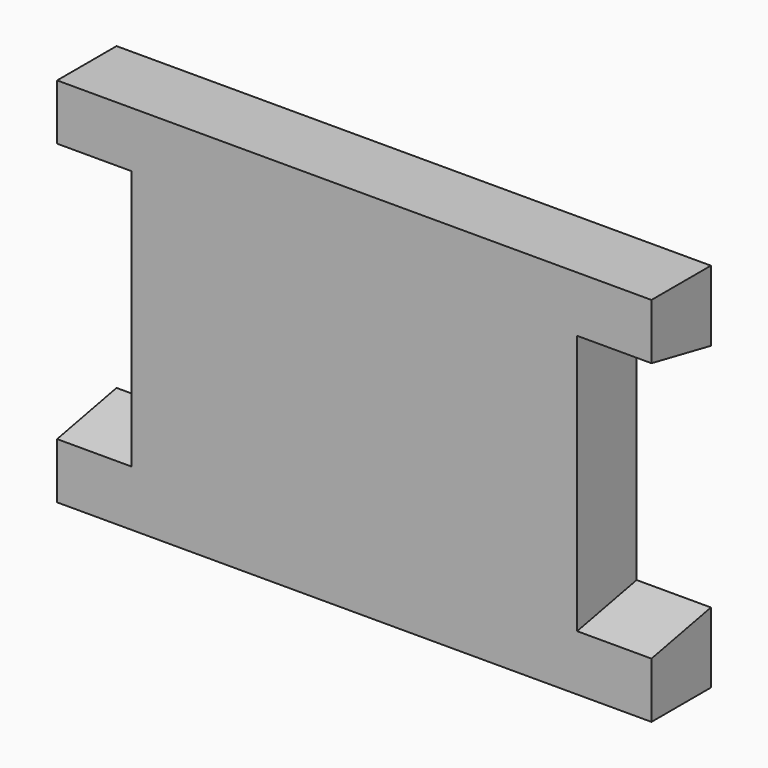
from build123d import *

# Parameters (mm, degrees)
F0_W     = 12.7
F0_H     = 63.5
F1_DEPTH = 50.8
F3_DEPTH = 12.7


# Not quite as in the source:
# - a pattern or mirror of a feature is missing from the dataset's text; its kind, count and spacing are read off the source's solid


with BuildPart() as f1:
    # F0 (on Right) → F1 (new body, symmetric)
    with BuildSketch(Plane.YZ):
        Rectangle(F0_W, F0_H)
    extrude(amount=F1_DEPTH, both=True)

    # F2 (on face) → F3 (cut)
    with BuildSketch(Plane(origin=(-50.8, 0, 0), x_dir=(0, -1, 0), z_dir=(-1, 0, 0))):
        Polygon((6.35, -22.225), (6.35, 22.225), (-6.35, 19.6872895852), (-6.35, -19.6872895852), align=None)
    f3 = extrude(amount=-F3_DEPTH, mode=Mode.SUBTRACT)

    # F3_copies: F3 across plane
    add(f3.mirror(Plane(origin=(0, 0, 0), x_dir=(0, 0, 1), z_dir=(1, 0, 0))), mode=Mode.SUBTRACT)


solid = f1.part
